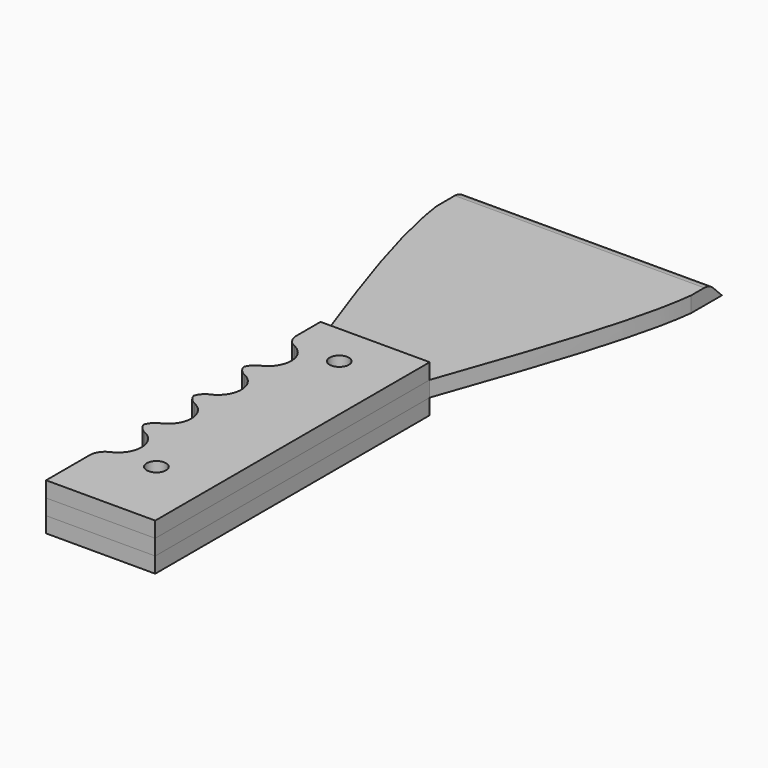
from build123d import *

# Parameters (mm, degrees)
F0_W          = 35
F0_H          = 90
F0_H_2        = 110
F1_DEPTH      = 5
F2_W          = 35
F2_H          = 110
F4_DEPTH      = 5
F3_W          = 35
F3_H          = 110
F5_DEPTH      = 5
F7_DEPTH      = 25
F6_R          = 7.5
F8_DEPTH      = 25
F9_T1_DEPTH   = 24.7821961869
F9_2_T1_DEPTH = 24.7821961869
F9_3_T1_DEPTH = 24.7821961869
F10_R         = 3.1
F11_DEPTH     = 25
F12_DEPTH     = 25
F13_T1_DEPTH  = 110.8601958556
F14_R         = 5


# Not quite as in the source:
# - a fillet or chamfer that OpenCascade refuses, or shapes differently, is made with other operations: its cross-section is extruded or revolved along the edge and cut away or added


with BuildPart() as f1:
    # F0 (on Top) → F1 (new body)
    with BuildSketch(Plane.XY):
        with BuildLine():
            add(Edge.make_bspline(
                [(-4.864667505, 41.1189725995), (-14.8268111493, 68.8529683822), (-24.7889547935, 96.5869641649), (-27.364667505, 115.7758631074)],
                knots=[0, 0, 0, 0, 0.5211248606, 0.5211248606, 0.5211248606, 0.5211248606], degree=3))
            Line((-4.864667505, 41.1189725995), (-4.864667505, 131.1189725995))
            Line((-4.864667505, 131.1189725995), (-27.364667505, 131.1189725995))
            Line((-27.364667505, 131.1189725995), (-27.364667505, 115.7758631074))
        make_face()
        with Locations((12.635332495, 86.1189725995)):
            Rectangle(F0_W, F0_H)
        with BuildLine():
            Line((30.135332495, 131.1189725995), (30.135332495, 41.1189725995))
            add(Edge.make_bspline(
                [(30.135332495, 41.1189725995), (40.232951817, 69.7853589458), (50.330571139, 98.4517452921), (52.635332495, 117.7113411352)],
                knots=[0, 0, 0, 0, 0.5432365903, 0.5432365903, 0.5432365903, 0.5432365903], degree=3))
            Line((52.635332495, 117.7113411352), (52.635332495, 131.1189725995))
            Line((52.635332495, 131.1189725995), (30.135332495, 131.1189725995))
        make_face()
        with Locations((12.635332495, -13.8810274005)):
            Rectangle(F0_W, F0_H_2)
    extrude(amount=F1_DEPTH)


with BuildPart() as f4:
    # F2 (on face) → F4 (new body)
    with BuildSketch(Plane.XY.offset(5)):
        with Locations((12.635332495, -13.8810274005)):
            Rectangle(F2_W, F2_H)
    extrude(amount=F4_DEPTH)


with BuildPart() as f5:
    # F3 (on face) → F5 (new body)
    with BuildSketch(Plane(origin=(0, 0, 0), x_dir=(1, 0, 0), z_dir=(0, 0, -1))):
        with Locations((12.635332495, 13.8810274005)):
            Rectangle(F3_W, F3_H)
    extrude(amount=F5_DEPTH)


with BuildPart() as f7_tool:
    # F6 (on face) → F7 (new body)
    with BuildSketch(Plane.XY.offset(10)):
        with BuildLine():
            ThreePointArc((-4.864667505, 12.5), (0.4386333539, 14.6966991411), (2.635332495, 20))
            ThreePointArc((2.635332495, 20), (0.4386333539, 25.3033008589), (-4.864667505, 27.5))
            Line((-4.864667505, 27.5), (-4.864667505, 12.5))
        make_face()
    extrude(amount=-F7_DEPTH)


with BuildPart() as f1_1:
    add(f1.part)

    # F7: cut by f7_tool
    add(f7_tool.part, mode=Mode.SUBTRACT)


with BuildPart() as f4_1:
    add(f4.part)

    # F7: cut by f7_tool
    add(f7_tool.part, mode=Mode.SUBTRACT)


with BuildPart() as f5_1:
    add(f5.part)

    # F7: cut by f7_tool
    add(f7_tool.part, mode=Mode.SUBTRACT)


with BuildPart() as f8_tool:
    # F6 (on face) → F8 (new body)
    with BuildSketch(Plane.XY.offset(10)):
        with Locations((-4.864667505, 20)):
            Circle(F6_R)
        with Locations((-4.864667505, 0)):
            Circle(F6_R)
        with Locations((-4.864667505, -20)):
            Circle(F6_R)
        with Locations((-4.864667505, -40)):
            Circle(F6_R)
    extrude(amount=-F8_DEPTH)


with BuildPart() as f1_2:
    add(f1_1.part)

    # F8: cut by f8_tool
    add(f8_tool.part, mode=Mode.SUBTRACT)

    # F9: fillet of radius 5 on 8 edges, made by hand

    # F9_s2 → F9_t1 (cut)
    with BuildSketch(Plane.XY.offset(-9.8910980935)):
        with BuildLine():
            ThreePointArc((-1.864667505, 26.8738635424), (-4.0479676377, 28.7178264499), (-4.864667505, 31.4564392374))
            Line((-4.864667505, 31.4564392374), (-4.864667505, 27.5))
            ThreePointArc((-4.864667505, 27.5), (-3.3323451774, 27.341797347), (-1.864667505, 26.8738635424))
        make_face()
        with BuildLine():
            ThreePointArc((-1.864667505, 13.1261364576), (-4.0479676377, 11.2821735501), (-4.864667505, 8.5435607626))
            Line((-4.864667505, 8.5435607626), (-4.864667505, 12.5))
            ThreePointArc((-4.864667505, 12.5), (-3.3323451774, 12.658202653), (-1.864667505, 13.1261364576))
        make_face()
        with BuildLine():
            ThreePointArc((-4.864667505, 11.4564392374), (-4.0479676377, 8.7178264499), (-1.864667505, 6.8738635424))
            ThreePointArc((-1.864667505, 6.8738635424), (-3.3323451774, 7.341797347), (-4.864667505, 7.5))
            Line((-4.864667505, 7.5), (-4.864667505, 11.4564392374))
        make_face()
        with BuildLine():
            ThreePointArc((-1.864667505, -6.8738635424), (-4.0479676377, -8.7178264499), (-4.864667505, -11.4564392374))
            Line((-4.864667505, -11.4564392374), (-4.864667505, -7.5))
            ThreePointArc((-4.864667505, -7.5), (-3.3323451774, -7.341797347), (-1.864667505, -6.8738635424))
        make_face()
        with BuildLine():
            ThreePointArc((-4.864667505, -8.5435607626), (-4.0479676377, -11.2821735501), (-1.864667505, -13.1261364576))
            ThreePointArc((-1.864667505, -13.1261364576), (-3.3323451774, -12.658202653), (-4.864667505, -12.5))
            Line((-4.864667505, -12.5), (-4.864667505, -8.5435607626))
        make_face()
        with BuildLine():
            ThreePointArc((-1.864667505, -26.8738635424), (-4.0479676377, -28.7178264499), (-4.864667505, -31.4564392374))
            Line((-4.864667505, -31.4564392374), (-4.864667505, -27.5))
            ThreePointArc((-4.864667505, -27.5), (-3.3323451774, -27.341797347), (-1.864667505, -26.8738635424))
        make_face()
        with BuildLine():
            ThreePointArc((-4.864667505, -28.5435607626), (-4.0479676377, -31.2821735501), (-1.864667505, -33.1261364576))
            ThreePointArc((-1.864667505, -33.1261364576), (-3.3323451774, -32.658202653), (-4.864667505, -32.5))
            Line((-4.864667505, -32.5), (-4.864667505, -28.5435607626))
        make_face()
        with BuildLine():
            ThreePointArc((-1.864667505, -46.8738635424), (-4.0479676377, -48.7178264499), (-4.864667505, -51.4564392374))
            Line((-4.864667505, -51.4564392374), (-4.864667505, -47.5))
            ThreePointArc((-4.864667505, -47.5), (-3.3323451774, -47.341797347), (-1.864667505, -46.8738635424))
        make_face()
    extrude(amount=F9_T1_DEPTH, mode=Mode.SUBTRACT)


with BuildPart() as f4_2:
    add(f4_1.part)

    # F8: cut by f8_tool
    add(f8_tool.part, mode=Mode.SUBTRACT)

    # F9#2: fillet of radius 5 on 8 edges, made by hand

    # F9_2_s2 → F9_2_t1 (cut)
    with BuildSketch(Plane.XY.offset(-4.8910980935)):
        with BuildLine():
            ThreePointArc((-1.864667505, 26.8738635424), (-4.0479676377, 28.7178264499), (-4.864667505, 31.4564392374))
            Line((-4.864667505, 31.4564392374), (-4.864667505, 27.5))
            ThreePointArc((-4.864667505, 27.5), (-3.3323451774, 27.341797347), (-1.864667505, 26.8738635424))
        make_face()
        with BuildLine():
            ThreePointArc((-4.864667505, 8.5435607626), (-4.0479676377, 11.2821735501), (-1.864667505, 13.1261364576))
            ThreePointArc((-1.864667505, 13.1261364576), (-3.3323451774, 12.658202653), (-4.864667505, 12.5))
            Line((-4.864667505, 12.5), (-4.864667505, 8.5435607626))
        make_face()
        with BuildLine():
            ThreePointArc((-4.864667505, -11.4564392374), (-4.0479676377, -8.7178264499), (-1.864667505, -6.8738635424))
            ThreePointArc((-1.864667505, -6.8738635424), (-3.3323451774, -7.341797347), (-4.864667505, -7.5))
            Line((-4.864667505, -7.5), (-4.864667505, -11.4564392374))
        make_face()
        with BuildLine():
            ThreePointArc((-1.864667505, 6.8738635424), (-4.0479676377, 8.7178264499), (-4.864667505, 11.4564392374))
            Line((-4.864667505, 11.4564392374), (-4.864667505, 7.5))
            ThreePointArc((-4.864667505, 7.5), (-3.3323451774, 7.341797347), (-1.864667505, 6.8738635424))
        make_face()
        with BuildLine():
            ThreePointArc((-4.864667505, -31.4564392374), (-4.0479676377, -28.7178264499), (-1.864667505, -26.8738635424))
            ThreePointArc((-1.864667505, -26.8738635424), (-3.3323451774, -27.341797347), (-4.864667505, -27.5))
            Line((-4.864667505, -27.5), (-4.864667505, -31.4564392374))
        make_face()
        with BuildLine():
            ThreePointArc((-1.864667505, -13.1261364576), (-4.0479676377, -11.2821735501), (-4.864667505, -8.5435607626))
            Line((-4.864667505, -8.5435607626), (-4.864667505, -12.5))
            ThreePointArc((-4.864667505, -12.5), (-3.3323451774, -12.658202653), (-1.864667505, -13.1261364576))
        make_face()
        with BuildLine():
            ThreePointArc((-4.864667505, -51.4564392374), (-4.0479676377, -48.7178264499), (-1.864667505, -46.8738635424))
            ThreePointArc((-1.864667505, -46.8738635424), (-3.3323451774, -47.341797347), (-4.864667505, -47.5))
            Line((-4.864667505, -47.5), (-4.864667505, -51.4564392374))
        make_face()
        with BuildLine():
            ThreePointArc((-1.864667505, -33.1261364576), (-4.0479676377, -31.2821735501), (-4.864667505, -28.5435607626))
            Line((-4.864667505, -28.5435607626), (-4.864667505, -32.5))
            ThreePointArc((-4.864667505, -32.5), (-3.3323451774, -32.658202653), (-1.864667505, -33.1261364576))
        make_face()
    extrude(amount=F9_2_T1_DEPTH, mode=Mode.SUBTRACT)


with BuildPart() as f5_2:
    add(f5_1.part)

    # F8: cut by f8_tool
    add(f8_tool.part, mode=Mode.SUBTRACT)

    # F9#3: fillet of radius 5 on 8 edges, made by hand

    # F9_3_s2 → F9_3_t1 (cut)
    with BuildSketch(Plane.XY.offset(-14.8910980935)):
        with BuildLine():
            ThreePointArc((-4.864667505, 31.4564392374), (-4.0479676377, 28.7178264499), (-1.864667505, 26.8738635424))
            ThreePointArc((-1.864667505, 26.8738635424), (-3.3323451774, 27.341797347), (-4.864667505, 27.5))
            Line((-4.864667505, 27.5), (-4.864667505, 31.4564392374))
        make_face()
        with BuildLine():
            ThreePointArc((-1.864667505, 13.1261364576), (-4.0479676377, 11.2821735501), (-4.864667505, 8.5435607626))
            Line((-4.864667505, 8.5435607626), (-4.864667505, 12.5))
            ThreePointArc((-4.864667505, 12.5), (-3.3323451774, 12.658202653), (-1.864667505, 13.1261364576))
        make_face()
        with BuildLine():
            ThreePointArc((-4.864667505, 11.4564392374), (-4.0479676377, 8.7178264499), (-1.864667505, 6.8738635424))
            ThreePointArc((-1.864667505, 6.8738635424), (-3.3323451774, 7.341797347), (-4.864667505, 7.5))
            Line((-4.864667505, 7.5), (-4.864667505, 11.4564392374))
        make_face()
        with BuildLine():
            ThreePointArc((-1.864667505, -6.8738635424), (-4.0479676377, -8.7178264499), (-4.864667505, -11.4564392374))
            Line((-4.864667505, -11.4564392374), (-4.864667505, -7.5))
            ThreePointArc((-4.864667505, -7.5), (-3.3323451774, -7.341797347), (-1.864667505, -6.8738635424))
        make_face()
        with BuildLine():
            ThreePointArc((-4.864667505, -8.5435607626), (-4.0479676377, -11.2821735501), (-1.864667505, -13.1261364576))
            ThreePointArc((-1.864667505, -13.1261364576), (-3.3323451774, -12.658202653), (-4.864667505, -12.5))
            Line((-4.864667505, -12.5), (-4.864667505, -8.5435607626))
        make_face()
        with BuildLine():
            ThreePointArc((-1.864667505, -26.8738635424), (-4.0479676377, -28.7178264499), (-4.864667505, -31.4564392374))
            Line((-4.864667505, -31.4564392374), (-4.864667505, -27.5))
            ThreePointArc((-4.864667505, -27.5), (-3.3323451774, -27.341797347), (-1.864667505, -26.8738635424))
        make_face()
        with BuildLine():
            ThreePointArc((-4.864667505, -51.4564392374), (-4.0479676377, -48.7178264499), (-1.864667505, -46.8738635424))
            ThreePointArc((-1.864667505, -46.8738635424), (-3.3323451774, -47.341797347), (-4.864667505, -47.5))
            Line((-4.864667505, -47.5), (-4.864667505, -51.4564392374))
        make_face()
        with BuildLine():
            ThreePointArc((-4.864667505, -28.5435607626), (-4.0479676377, -31.2821735501), (-1.864667505, -33.1261364576))
            ThreePointArc((-1.864667505, -33.1261364576), (-3.3323451774, -32.658202653), (-4.864667505, -32.5))
            Line((-4.864667505, -32.5), (-4.864667505, -28.5435607626))
        make_face()
    extrude(amount=F9_3_T1_DEPTH, mode=Mode.SUBTRACT)


with BuildPart() as f11_tool:
    # F10 (on face) → F11 (new body)
    with BuildSketch(Plane.XY.offset(10)):
        with Locations((12.1272588149, 27.3931510746)):
            Circle(F10_R)
    extrude(amount=-F11_DEPTH)


with BuildPart() as f1_3:
    add(f1_2.part)

    # F11: cut by f11_tool
    add(f11_tool.part, mode=Mode.SUBTRACT)


with BuildPart() as f4_3:
    add(f4_2.part)

    # F11: cut by f11_tool
    add(f11_tool.part, mode=Mode.SUBTRACT)


with BuildPart() as f5_3:
    add(f5_2.part)

    # F11: cut by f11_tool
    add(f11_tool.part, mode=Mode.SUBTRACT)


with BuildPart() as f12_tool:
    # F10 (on face) → F12 (new body)
    with BuildSketch(Plane.XY.offset(10)):
        with Locations((12.1272588149, 27.3931510746)):
            Circle(F10_R)
        with Locations((12.1272588149, -45.9034666419)):
            Circle(F10_R)
    extrude(amount=-F12_DEPTH)


with BuildPart() as f1_4:
    add(f1_3.part)

    # F12: cut by f12_tool
    add(f12_tool.part, mode=Mode.SUBTRACT)

    # F13: chamfer of 6 on 1 edges, made by hand

    # F13_s2 → F13_t1 (cut)
    with BuildSketch(Plane.YZ.offset(-42.7947654328)):
        Polygon((125.1189725995, 5), (131.1189725995, -1), (131.1189725995, 5), align=None)
    extrude(amount=F13_T1_DEPTH, mode=Mode.SUBTRACT)

    # F14
    f14_edges = [f1_4.edges().sort_by_distance(p)[0] for p in [
        (12.635332, 125.118973, 5),
    ]]
    fillet(f14_edges, radius=F14_R)


with BuildPart() as f4_4:
    add(f4_3.part)

    # F12: cut by f12_tool
    add(f12_tool.part, mode=Mode.SUBTRACT)


with BuildPart() as f5_4:
    add(f5_3.part)

    # F12: cut by f12_tool
    add(f12_tool.part, mode=Mode.SUBTRACT)


solid = Compound([f1_4.part, f4_4.part, f5_4.part])
